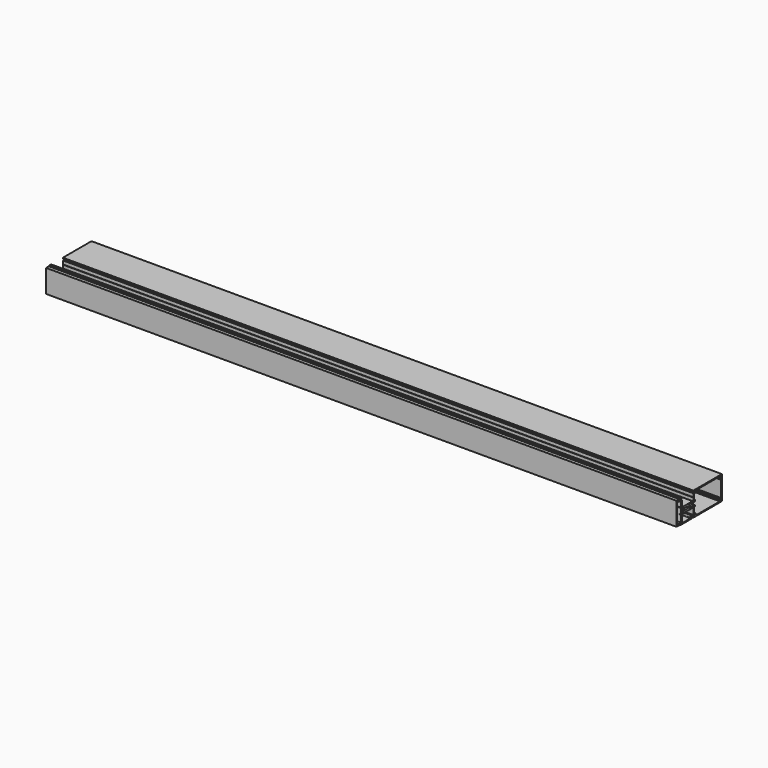
from build123d import *

# Parameters (mm, degrees)
F1_DEPTH = 1676.4
F2_DEPTH = 1676.4


# Not quite as in the source:
# - ends of sketch curves that miss each other by under 0.0002 mm in the source are joined


with BuildPart() as f1:
    # F0 (on Right) → F1 (new body)
    with BuildSketch(Plane.YZ):
        with BuildLine():
            Line((70.9422, -57.3056004), (70.9422, -51.9208004))
            Line((70.9422, -51.9208004), (71.755, -51.9208004))
            Line((71.755, -51.9208004), (70.075425, -49.011713))
            ThreePointArc((70.075425, -49.011713), (69.9365522187, -48.8728127332), (69.7468252, -48.821975))
            Line((69.7468252, -48.821975), (63.0174, -48.8220004))
            Line((63.0174, -48.8220004), (63.0174, -50.3968004))
            Line((63.0174, -50.3968004), (69.3674, -50.3968004))
            Line((69.3674, -50.3968004), (69.3674, -57.5596004))
            Line((69.3674, -57.5596004), (-8.2296, -57.5596004))
            Line((-8.2296, -57.5596004), (-8.2296, -56.2896004))
            ThreePointArc((-8.2296, -56.2896004), (-8.6759692655, -55.2119696655), (-9.7536, -54.7656004))
            Line((-9.7536, -54.7656004), (-11.7856, -54.7656004))
            ThreePointArc((-11.7856, -54.7656004), (-12.5476, -55.5276004), (-11.7856, -56.2896004))
            Line((-11.7856, -56.2896004), (-9.8806, -56.2896004))
            Line((-9.8806, -56.2896004), (-9.8245814443, -56.294824928))
            Line((-9.8245814443, -56.294824928), (-9.8449373618, -58.3216004))
            Line((-9.8449373618, -58.3216004), (-9.8806, -58.3216004))
            Line((-9.8806, -58.3216004), (-12.0396, -58.3216004))
            ThreePointArc((-12.0396, -58.3216004), (-12.3988102448, -58.4703901552), (-12.5476, -58.8296004))
            Line((-12.5476, -58.8296004), (-12.5476, -59.8456004))
            Line((-12.5476, -59.8456004), (75.4107966, -59.8456004))
            ThreePointArc((75.4107966, -59.8456004), (75.6454620013, -59.6888019918), (75.5904017224, -59.4119952776))
            Line((75.5904017224, -59.4119952776), (73.4840034, -57.3056004))
            Line((73.4840034, -57.3056004), (70.9422, -57.3056004))
        make_face()
        with BuildLine():
            Line((-19.05, -2.8988004), (-19.05, -10.6331004))
            Line((-19.05, -10.6331004), (-19.05, -11.8396004))
            Line((-19.05, -11.8396004), (-18.669, -12.2206004))
            Line((-18.669, -12.2206004), (-19.05, -12.6016004))
            Line((-19.05, -12.6016004), (-19.05, -21.4154004))
            ThreePointArc((-19.05, -21.4154004), (-19.1243948776, -21.5950055224), (-19.304, -21.6694004))
            Line((-19.304, -21.6694004), (-20.7264, -21.6694004))
            ThreePointArc((-20.7264, -21.6694004), (-20.9060051224, -21.5950055224), (-20.9804, -21.4154004))
            Line((-20.9804, -21.4154004), (-20.9804, -20.3994004))
            ThreePointArc((-20.9804, -20.3994004), (-21.0547948776, -20.2197952776), (-21.2344, -20.1454004))
            Line((-21.2344, -20.1454004), (-22.225, -20.1454004))
            Line((-22.225, -20.1454004), (-31.75, -20.1454004))
            Line((-31.75, -20.1454004), (-41.275, -20.1454004))
            Line((-41.275, -20.1454004), (-50.8, -20.1454004))
            Line((-50.8, -20.1454004), (-50.8, -21.1614004))
            Line((-50.8, -21.1614004), (-51.181, -21.5424004))
            Line((-51.181, -21.5424004), (-50.8, -21.9234004))
            Line((-50.8, -21.9234004), (-50.8, -23.7776004))
            Line((-50.8, -23.7776004), (-51.181, -24.1586004))
            Line((-51.181, -24.1586004), (-50.8, -24.5396004))
            Line((-50.8, -24.5396004), (-50.8, -25.5556004))
            Line((-50.8, -25.5556004), (-39.878, -25.5556004))
            Line((-39.878, -25.5556004), (-34.3379552, -27.0400526))
            ThreePointArc((-34.3379552, -27.0400526), (-33.528, -28.0956004), (-34.3379547374, -29.1511499265))
            Line((-34.3379547374, -29.1511499265), (-39.878, -30.6356004))
            Line((-39.878, -30.6356004), (-50.8, -30.6356004))
            Line((-50.8, -30.6356004), (-50.8, -31.6516004))
            Line((-50.8, -31.6516004), (-51.181, -32.0326004))
            Line((-51.181, -32.0326004), (-50.8, -32.4136004))
            Line((-50.8, -32.4136004), (-50.8, -34.2678004))
            Line((-50.8, -34.2678004), (-51.181, -34.6488004))
            Line((-51.181, -34.6488004), (-50.8, -35.0298004))
            Line((-50.8, -35.0298004), (-50.8, -36.0458004))
            Line((-50.8, -36.0458004), (-21.2344, -36.0458004))
            ThreePointArc((-21.2344, -36.0458004), (-21.0547948776, -35.9714055224), (-20.9804, -35.7918004))
            Line((-20.9804, -35.7918004), (-20.9804, -34.7758004))
            ThreePointArc((-20.9804, -34.7758004), (-20.9060051224, -34.5961952776), (-20.7264, -34.5218004))
            Line((-20.7264, -34.5218004), (-19.304, -34.5218004))
            ThreePointArc((-19.304, -34.5218004), (-19.1243948776, -34.5961952776), (-19.05, -34.7758004))
            Line((-19.05, -34.7758004), (-19.05, -53.2924004))
            ThreePointArc((-19.05, -53.2924004), (-18.8142213914, -53.6446385971), (-18.3987047377, -53.5609175711))
            ThreePointArc((-18.3987047377, -53.5609175711), (-17.6552346218, -53.0614614802), (-16.7769286, -52.8860004))
            Line((-16.7769286, -52.8860004), (-16.51, -52.8860004))
            ThreePointArc((-16.51, -52.8860004), (-15.6119743879, -53.2579747879), (-15.24, -54.1560004))
            Line((-15.24, -54.1560004), (-15.24, -56.3912004))
            ThreePointArc((-15.24, -56.3912004), (-15.6119743879, -57.2892260121), (-16.51, -57.6612004))
            Line((-16.51, -57.6612004), (-16.7769286, -57.6612004))
            ThreePointArc((-16.7769286, -57.6612004), (-17.6552346218, -57.4857393198), (-18.3987125392, -56.9862909792))
            ThreePointArc((-18.3987125392, -56.9862909792), (-18.8142213914, -56.9025622029), (-19.05, -57.2548004))
            Line((-19.05, -57.2548004), (-19.05, -59.3376004))
            ThreePointArc((-19.05, -59.3376004), (-18.9012102448, -59.6968106448), (-18.542, -59.8456004))
            Line((-18.542, -59.8456004), (-13.208, -59.8456004))
            ThreePointArc((-13.208, -59.8456004), (-12.8487897552, -59.6968106448), (-12.7, -59.3376004))
            Line((-12.7, -59.3376004), (-12.7, -58.0676004))
            Line((-12.7, -58.0676004), (-10.6426, -58.0676004))
            ThreePointArc((-10.6426, -58.0676004), (-9.8806, -57.3056004), (-10.6426, -56.5436004))
            Line((-10.6426, -56.5436004), (-12.7, -56.5436004))
            Line((-12.7, -56.5436004), (-12.7, -51.3366004))
            ThreePointArc((-12.7, -51.3366004), (-12.8487897552, -50.9773901552), (-13.208, -50.8286004))
            Line((-13.208, -50.8286004), (-15.875, -50.8286004))
            Line((-15.875, -50.8286004), (-15.875, -36.0458004))
            Line((-15.875, -36.0458004), (-13.462, -36.0458004))
            ThreePointArc((-13.462, -36.0458004), (-12.9231846327, -35.8226157673), (-12.7, -35.2838004))
            Line((-12.7, -35.2838004), (-12.7, -33.6328004))
            ThreePointArc((-12.7, -33.6328004), (-12.9231846327, -33.0939850327), (-13.462, -32.8708004))
            Line((-13.462, -32.8708004), (-15.875, -32.8708004))
            ThreePointArc((-15.875, -32.8708004), (-16.3213692655, -31.7931696655), (-17.399, -31.3468004))
            Line((-17.399, -31.3468004), (-22.6314, -31.3468004))
            ThreePointArc((-22.6314, -31.3468004), (-23.7090307345, -31.7931696655), (-24.1554, -32.8708004))
            Line((-24.1554, -32.8708004), (-32.476948, -32.8708004))
            ThreePointArc((-32.476948, -32.8708004), (-32.9712512757, -32.4799681072), (-32.7049652499, -31.9088487134))
            ThreePointArc((-32.7049652499, -31.9088487134), (-30.353, -28.0956004), (-32.7049647769, -24.2823511451))
            ThreePointArc((-32.7049647769, -24.2823511451), (-32.9712512757, -23.7112326928), (-32.476948, -23.3204004))
            Line((-32.476948, -23.3204004), (-24.1554, -23.3204004))
            ThreePointArc((-24.1554, -23.3204004), (-23.7090307345, -24.3980311345), (-22.6314, -24.8444004))
            Line((-22.6314, -24.8444004), (-17.399, -24.8444004))
            ThreePointArc((-17.399, -24.8444004), (-16.3213692655, -24.3980311345), (-15.875, -23.3204004))
            Line((-15.875, -23.3204004), (-13.462, -23.3204004))
            ThreePointArc((-13.462, -23.3204004), (-12.9231846327, -23.0972157673), (-12.7, -22.5584004))
            Line((-12.7, -22.5584004), (-12.7, -20.9074004))
            ThreePointArc((-12.7, -20.9074004), (-12.9231846327, -20.3685850327), (-13.462, -20.1454004))
            Line((-13.462, -20.1454004), (-15.875, -20.1454004))
            Line((-15.875, -20.1454004), (-15.875, -5.3626004))
            Line((-15.875, -5.3626004), (-13.208, -5.3626004))
            Line((-13.208, -5.3626004), (-12.7, -4.8546004))
            Line((-12.7, -4.8546004), (-12.7, 0.3523996))
            ThreePointArc((-12.7, 0.3523996), (-12.4768153673, 0.8912149673), (-11.938, 1.1143996))
            Line((-11.938, 1.1143996), (72.263, 1.1143996))
            ThreePointArc((72.263, 1.1143996), (72.8018153673, 0.8912149673), (73.025, 0.3523996))
            Line((73.025, 0.3523996), (73.025, -2.9496004))
            ThreePointArc((73.025, -2.9496004), (72.5786307345, -4.0272311345), (71.501, -4.4736004))
            Line((71.501, -4.4736004), (70.612, -4.4736004))
            Line((70.612, -4.4736004), (70.612, -7.6486004))
            Line((70.612, -7.6486004), (71.501, -7.6486004))
            ThreePointArc((71.501, -7.6486004), (72.5786307345, -8.0949696655), (73.025, -9.1726004))
            Line((73.025, -9.1726004), (73.025, -51.1588004))
            ThreePointArc((73.025, -51.1588004), (72.8018153673, -51.6976157673), (72.263, -51.9208004))
            Line((72.263, -51.9208004), (71.755, -51.9208004))
            Line((71.755, -51.9208004), (70.9422, -51.9208004))
            Line((70.9422, -51.9208004), (72.3676734, -55.8373026))
            Line((72.3676734, -55.8373026), (75.7663966, -59.2360004))
            ThreePointArc((75.7663966, -59.2360004), (76.0432015918, -59.2910624013), (76.2, -59.056397))
            Line((76.2, -59.056397), (76.2, 3.6543996))
            Line((76.2, 3.6543996), (-18.542, 3.6543996))
            ThreePointArc((-18.542, 3.6543996), (-18.9012102448, 3.5056098448), (-19.05, 3.1463996))
            Line((-19.05, 3.1463996), (-19.05, 1.0635996))
            ThreePointArc((-19.05, 1.0635996), (-18.8142213914, 0.7113614029), (-18.3987047377, 0.7950824289))
            ThreePointArc((-18.3987047377, 0.7950824289), (-17.6552346218, 1.2945385198), (-16.7769286, 1.4699996))
            Line((-16.7769286, 1.4699996), (-16.51, 1.4699996))
            ThreePointArc((-16.51, 1.4699996), (-15.6119743879, 1.0980252121), (-15.24, 0.1999996))
            Line((-15.24, 0.1999996), (-15.24, -2.0352004))
            ThreePointArc((-15.24, -2.0352004), (-15.6119743879, -2.9332260121), (-16.51, -3.3052004))
            Line((-16.51, -3.3052004), (-16.7769286, -3.3052004))
            ThreePointArc((-16.7769286, -3.3052004), (-17.6552346218, -3.1297393198), (-18.3987125392, -2.6302909792))
            ThreePointArc((-18.3987125392, -2.6302909792), (-18.8142213914, -2.5465622029), (-19.05, -2.8988004))
        make_face()
    extrude(amount=F1_DEPTH)


with BuildPart() as f1b:
    # F0 (on Right) → F1, piece 2 (new body)
    with BuildSketch(Plane.YZ):
        with BuildLine():
            ThreePointArc((-65.6176205987, 1.4700005462), (-65.1549312963, 0.8446470138), (-64.4144, 0.6063996))
            ThreePointArc((-64.4144, 0.6063996), (-65.1328204897, 0.9039791103), (-65.4304, 1.6223996))
            Line((-65.4304, 1.6223996), (-65.4304, 2.3843996))
            Line((-65.4304, 2.3843996), (-74.676, 2.3843996))
            Line((-74.676, 2.3843996), (-74.676, -58.5756004))
            Line((-74.676, -58.5756004), (-65.4304, -58.5756004))
            Line((-65.4304, -58.5756004), (-65.4304, -57.8136004))
            ThreePointArc((-65.4304, -57.8136004), (-65.1328204897, -57.0951799103), (-64.4144, -56.7976004))
            ThreePointArc((-64.4144, -56.7976004), (-63.5163743879, -57.1695747879), (-63.1444, -58.0676004))
            Line((-63.1444, -58.0676004), (-63.1444, -59.0836004))
            ThreePointArc((-63.1444, -59.0836004), (-62.9212153673, -59.6224157673), (-62.3824, -59.8456004))
            Line((-62.3824, -59.8456004), (-25.4, -59.8456004))
            Line((-25.4, -59.8456004), (-25.4, -50.4476004))
            ThreePointArc((-25.4, -50.4476004), (-25.6231846327, -49.9087850327), (-26.162, -49.6856004))
            Line((-26.162, -49.6856004), (-27.178, -49.6856004))
            ThreePointArc((-27.178, -49.6856004), (-27.7168153673, -49.9087850327), (-27.94, -50.4476004))
            Line((-27.94, -50.4476004), (-27.94, -55.7816004))
            ThreePointArc((-27.94, -55.7816004), (-28.3863692655, -56.8592311345), (-29.464, -57.3056004))
            Line((-29.464, -57.3056004), (-55.626, -57.3056004))
            ThreePointArc((-55.626, -57.3056004), (-56.7036307345, -56.8592311345), (-57.15, -55.7816004))
            Line((-57.15, -55.7816004), (-57.15, -36.0458004))
            Line((-57.15, -36.0458004), (-57.15, -34.4583004))
            Line((-57.15, -34.4583004), (-57.15, -33.8106004))
            Line((-57.15, -33.8106004), (-56.769, -33.4296004))
            Line((-56.769, -33.4296004), (-57.15, -33.0486004))
            Line((-57.15, -33.0486004), (-57.15, -31.4738004))
            Line((-57.15, -31.4738004), (-60.325, -31.4738004))
            Line((-60.325, -31.4738004), (-60.325, -35.7156004))
            Line((-60.325, -35.7156004), (-59.69, -36.3506004))
            Line((-59.69, -36.3506004), (-59.69, -54.7656004))
            Line((-59.69, -54.7656004), (-66.568955, -54.7656004))
            Line((-66.568955, -54.7656004), (-73.3418166637, -54.7656004))
            Line((-73.3418166637, -54.7656004), (-73.3418166637, -1.0101338848))
            Line((-73.3418166637, -1.0101338848), (-65.6176205987, 1.4700005462))
        make_face()
        with BuildLine():
            ThreePointArc((-63.1444, 1.8763996), (-63.5163743879, 0.9783739879), (-64.4144, 0.6063996))
            ThreePointArc((-64.4144, 0.6063996), (-65.1549312963, 0.8446470138), (-65.6176205987, 1.4700005462))
            Line((-65.6176205987, 1.4700005462), (-70.2564, -1.2082018))
            ThreePointArc((-70.2564, -1.2082018), (-70.6282817077, -2.5960833776), (-69.2403998224, -2.9679649077))
            Line((-69.2403998224, -2.9679649077), (-66.568955, -1.4256004))
            Line((-66.568955, -1.4256004), (-63.1444, -1.4256004))
            Line((-63.1444, -1.4256004), (-63.1444, -4.3212004))
            ThreePointArc((-63.1444, -4.3212004), (-62.6980307345, -5.3988311345), (-61.6204, -5.8452004))
            Line((-61.6204, -5.8452004), (-59.69, -5.8452004))
            Line((-59.69, -5.8452004), (-59.69, -19.8406004))
            Line((-59.69, -19.8406004), (-60.325, -20.4756004))
            Line((-60.325, -20.4756004), (-60.325, -24.7174004))
            Line((-60.325, -24.7174004), (-57.15, -24.7174004))
            Line((-57.15, -24.7174004), (-57.15, -23.1426004))
            Line((-57.15, -23.1426004), (-56.769, -22.7616004))
            Line((-56.769, -22.7616004), (-57.15, -22.3806004))
            Line((-57.15, -22.3806004), (-57.15, -21.7329004))
            Line((-57.15, -21.7329004), (-57.15, -20.1454004))
            Line((-57.15, -20.1454004), (-57.15, -2.8988004))
            ThreePointArc((-57.15, -2.8988004), (-57.3857868835, -2.5465587914), (-57.8013078782, -2.630295929))
            ThreePointArc((-57.8013078782, -2.630295929), (-58.5447907782, -3.1297393198), (-59.4230968, -3.3052004))
            Line((-59.4230968, -3.3052004), (-59.69, -3.3052004))
            ThreePointArc((-59.69, -3.3052004), (-60.5880256121, -2.9332260121), (-60.96, -2.0352004))
            Line((-60.96, -2.0352004), (-60.96, 0.1999996))
            ThreePointArc((-60.96, 0.1999996), (-60.5880256121, 1.0980252121), (-59.69, 1.4699996))
            Line((-59.69, 1.4699996), (-59.4230968, 1.4699996))
            ThreePointArc((-59.4230968, 1.4699996), (-58.5447907782, 1.2945385198), (-57.8013128608, 0.7950901792))
            ThreePointArc((-57.8013128608, 0.7950901792), (-57.3857868835, 0.7113579914), (-57.15, 1.0635996))
            Line((-57.15, 1.0635996), (-57.15, 3.1463996))
            ThreePointArc((-57.15, 3.1463996), (-57.2987897552, 3.5056098448), (-57.658, 3.6543996))
            Line((-57.658, 3.6543996), (-62.3824, 3.6543996))
            ThreePointArc((-62.3824, 3.6543996), (-62.9212153673, 3.4312149673), (-63.1444, 2.8923996))
            Line((-63.1444, 2.8923996), (-63.1444, 1.8763996))
        make_face()
    extrude(amount=F1_DEPTH)

    # F0 (on Right) → F2 (join)
    with BuildSketch(Plane.YZ):
        Polygon((-60.325, -28.4766004), (-60.325, -31.4738004), (-57.15, -31.4738004), (-57.15, -24.7174004), (-60.325, -24.7174004), (-60.325, -27.7146004), align=None)
    extrude(amount=F2_DEPTH)


solid = Compound([f1.part, f1b.part])
